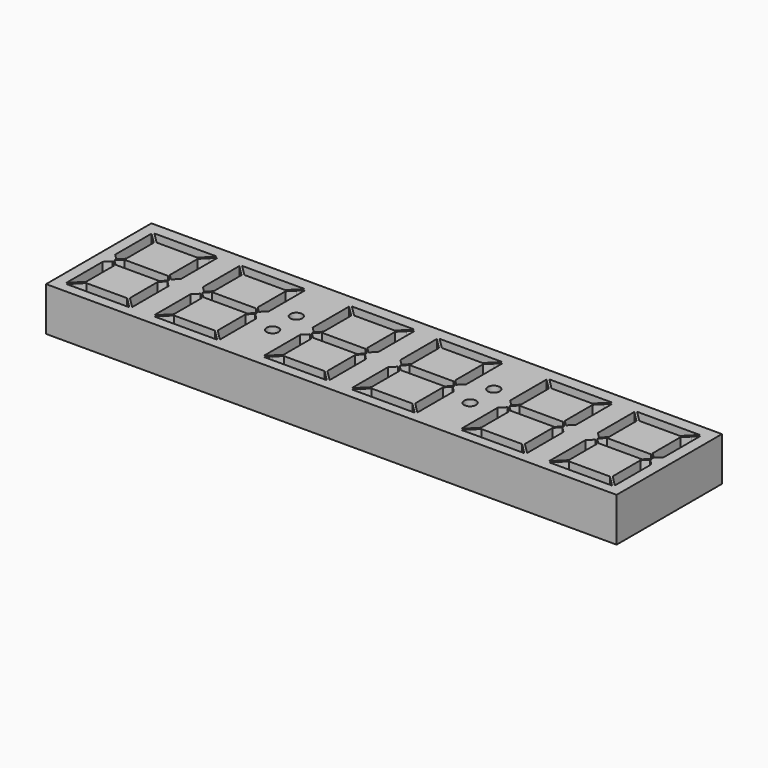
from build123d import *

# Parameters (mm, degrees)
F0_R     = 3.4648968079
F1_DEPTH = 25.4


# Not quite as in the source:
# - ends of sketch curves that miss each other by under 0.0002 mm in the source are joined


with BuildPart() as f1:
    # F0 (on Top) → F1 (new body)
    with BuildSketch(Plane.XY):
        Polygon((-45.9224169783, 52.1854245931), (-71.324658747, 52.1854245931), (-122.124658747, 52.1854245931), (-122.124658747, -24.0145754069), (-71.324658747, -24.0145754069), (-20.5201752096, -24.0145754069), (-7.824658747, -24.0145754069), (-7.8201752096, -24.0145754069), (42.975341253, -24.0145754069), (93.7798247904, -24.0145754069), (106.475341253, -24.0145754069), (106.4798247904, -24.0145754069), (157.275341253, -24.0145754069), (208.0798247904, -24.0145754069), (208.0798247904, 52.1854245931), (182.6775830217, 52.1854245931), (157.275341253, 52.1854245931), (106.4798247904, 52.1854245931), (106.475341253, 52.1854245931), (100.1298247904, 52.1854245931), (93.7798247904, 52.1854245931), (68.3775830217, 52.1854245931), (42.975341253, 52.1854245931), (-7.8201752096, 52.1854245931), (-7.824658747, 52.1854245931), (-14.1701752096, 52.1854245931), (-20.5201752096, 52.1854245931), align=None)
        Polygon((-114.8766638426, -18.2225372752), (-112.1506766486, -15.4965500813), (-108.5266638426, -11.8725372752), (-84.9227150668, -11.8725372752), (-81.2987022607, -15.4965500813), (-78.5727150668, -18.2225372752), align=None, mode=Mode.SUBTRACT)
        Polygon((-27.7726536514, -18.2225372752), (-64.0766024272, -18.2225372752), (-61.3506152332, -15.4965500813), (-57.7266024272, -11.8725372752), (-34.1226536514, -11.8725372752), (-30.4986408454, -15.4965500813), align=None, mode=Mode.SUBTRACT)
        Polygon((5.7733361574, -11.8725372752), (29.3772849332, -11.8725372752), (33.0012977393, -15.4965500813), (35.7272849332, -18.2225372752), (-0.5766638426, -18.2225372752), (2.1493233514, -15.4965500813), align=None, mode=Mode.SUBTRACT)
        Polygon((-115.7770073018, 9.0053659809), (-115.7061190955, 9.0824627244), (-112.5653735672, 12.2574627244), (-109.4246280391, 9.0824627243), (-109.4246280391, -10.9745116633), (-113.0486408451, -14.5985244694), (-115.7746284012, -17.3245116571), align=None, mode=Mode.SUBTRACT)
        Polygon((-80.8810682654, 12.2546509709), (-77.7403227372, 9.0796509709), (-77.6718137934, 9.0101770152), (-77.6718137934, -17.3273234166), (-80.3978009873, -14.6013362227), (-84.0218137919, -10.977323417), (-84.0218137936, 9.0796509708), align=None, mode=Mode.SUBTRACT)
        Polygon((-58.6275037021, -10.977323417), (-62.2515165067, -14.6013362227), (-64.9775037006, -17.3273234166), (-64.9775037006, 9.0101770152), (-64.9089947568, 9.0796509709), (-61.7682492285, 12.2546509709), (-58.6275037004, 9.0796509708), align=None, mode=Mode.SUBTRACT)
        Polygon((-112.5824693266, 13.5446828527), (-109.4275024956, 16.6996496838), (-84.0275012359, 16.699648424), (-80.866894333, 13.5446981166), (-84.0218137936, 10.349650971), (-109.4218137935, 10.349650971), (-109.4246752935, 10.3524770633), (-109.4259061434, 10.3536926829), align=None, mode=Mode.SUBTRACT)
        Polygon((-61.782423161, 13.5446981166), (-58.6218162581, 16.699648424), (-33.2218162581, 16.699648424), (-30.0668481674, 13.5446828527), (-33.2246280392, 10.3524627245), (-33.2275037004, 10.349650971), (-58.6275037003, 10.349650971), align=None, mode=Mode.SUBTRACT)
        Polygon((-26.8746890928, -17.3245116571), (-29.6006766488, -14.5985244694), (-33.2246894549, -10.9745116633), (-33.2246894549, 9.0824627243), (-30.0839439267, 12.2574627244), (-26.9431983985, 9.0824627244), (-26.8723101921, 9.0053659809), align=None, mode=Mode.SUBTRACT)
        Polygon((1.7346264327, 12.2574627244), (4.8753719609, 9.0824627243), (4.8753719609, -10.9745116633), (1.2513591549, -14.5985244694), (-1.4746284012, -17.3245116571), (-1.4770073018, 9.0053659809), (-1.4061190955, 9.0824627244), align=None, mode=Mode.SUBTRACT)
        Polygon((30.2781862081, -10.977323417), (30.2781862064, 9.0796509708), (33.4189317346, 12.2546509709), (36.5596772628, 9.0796509709), (36.6281862066, 9.0101770152), (36.6281862066, -17.3273234166), (33.9021990127, -14.6013362227), align=None, mode=Mode.SUBTRACT)
        with Locations((-14.1746894548, 4.9483692275)):
            Circle(F0_R, mode=Mode.SUBTRACT)
        Polygon((1.6986249251, 13.524648424), (1.6963722036, 13.524648424), (1.6974989639, 13.5257747847), align=None, mode=Mode.SUBTRACT)
        Polygon((4.8724987641, 16.699648424), (30.2724987641, 16.699648424), (33.4160560732, 13.5617171963), (33.433105667, 13.5446981166), (33.4503257953, 13.5621060558), (33.4503719609, 13.5274627244), (33.4160560732, 13.5274627245), (30.2781862064, 10.349650971), (4.8781862065, 10.3496509707), (4.8753105452, 10.3524627245), (1.7175306734, 13.5446828527), align=None, mode=Mode.SUBTRACT)
        Polygon((52.9493847668, -15.4965500813), (56.5733975728, -11.8725372752), (80.1773463486, -11.8725372752), (83.8013591546, -15.4965500813), (86.5273463486, -18.2225372752), (50.2233975728, -18.2225372752), align=None, mode=Mode.SUBTRACT)
        Polygon((120.0733361574, -11.8725372752), (143.6772849332, -11.8725372752), (147.3012977393, -15.4965500813), (150.0272849332, -18.2225372752), (113.7233361574, -18.2225372752), (116.4493233514, -15.4965500813), align=None, mode=Mode.SUBTRACT)
        Polygon((167.2493847668, -15.4965500813), (170.8733975728, -11.8725372752), (194.4773463486, -11.8725372752), (198.1013591546, -15.4965500813), (200.8273463486, -18.2225372752), (164.5233975728, -18.2225372752), align=None, mode=Mode.SUBTRACT)
        Polygon((52.5317507714, 12.2546509709), (55.6724962996, 9.0796509708), (55.6724962979, -10.977323417), (52.0484834933, -14.6013362227), (49.3224962994, -17.3273234166), (49.3224962994, 9.0101770152), (49.3910052432, 9.0796509709), align=None, mode=Mode.SUBTRACT)
        Polygon((81.0753105451, -10.9745116633), (81.0753105451, 9.0824627243), (84.2160560733, 12.2574627244), (87.3568016015, 9.0824627244), (87.4276898079, 9.0053659809), (87.4253109084, -17.3245116571), (84.6993233512, -14.5985244694), align=None, mode=Mode.SUBTRACT)
        Polygon((116.0346264327, 12.2574627244), (119.1753719609, 9.0824627243), (119.1753719609, -10.9745116633), (115.5513591549, -14.5985244694), (112.8253715988, -17.3245116571), (112.8229926982, 9.0053659809), (112.8938809045, 9.0824627244), align=None, mode=Mode.SUBTRACT)
        Polygon((81.0724962996, 10.3496509714), (55.6724962997, 10.3496509713), (52.5346109056, 13.5274473923), (52.5003105451, 13.5274627244), (52.5003567108, 13.5621060558), (52.517576839, 13.5446981166), (52.5346264328, 13.5617171963), (55.6781837419, 16.699648424), (81.0781837419, 16.699648424), (84.2331518326, 13.5446828527), (81.0753719608, 10.3524627245), align=None, mode=Mode.SUBTRACT)
        with Locations((100.1253105452, 4.9483692275)):
            Circle(F0_R, mode=Mode.SUBTRACT)
        Polygon((84.2531835421, 13.5257747847), (84.2543103024, 13.524648424), (84.252057581, 13.524648424), align=None, mode=Mode.SUBTRACT)
        Polygon((115.9986249251, 13.5246484235), (115.9963722036, 13.5246484235), (115.9974989639, 13.5257747847), align=None, mode=Mode.SUBTRACT)
        Polygon((144.5781862081, -10.977323417), (144.5781862064, 9.0796509708), (147.7189317346, 12.2546509709), (150.8596772628, 9.0796509709), (150.9281862066, 9.0101770152), (150.9281862066, -17.3273234166), (148.2021990127, -14.6013362227), align=None, mode=Mode.SUBTRACT)
        Polygon((166.8317507714, 12.2546509709), (169.9724962996, 9.0796509708), (169.9724962979, -10.977323417), (166.3484834933, -14.6013362227), (163.6224962994, -17.3273234166), (163.6224962994, 9.0101770152), (163.6910052432, 9.0796509709), align=None, mode=Mode.SUBTRACT)
        Polygon((195.3753105451, -10.9745116633), (195.3753105451, 9.0824627243), (198.5160560733, 12.2574627244), (201.6568016015, 9.0824627244), (201.7276898079, 9.0053659809), (201.7253109084, -17.3245116571), (198.9993233512, -14.5985244694), align=None, mode=Mode.SUBTRACT)
        Polygon((119.1724987641, 16.699648424), (144.5724987641, 16.699648424), (147.7160560732, 13.5617171963), (147.733105667, 13.5446981166), (147.7503257953, 13.5621060558), (147.7503719609, 13.5274627244), (147.7160560732, 13.5274627245), (144.5781862064, 10.349650971), (119.1781862065, 10.3496509704), (119.1753105452, 10.3524627245), (116.0175306734, 13.5446828527), align=None, mode=Mode.SUBTRACT)
        Polygon((195.3724962996, 10.3496509717), (169.9724962997, 10.3496509716), (166.8346109056, 13.5274473923), (166.8003105451, 13.5274627244), (166.8003567108, 13.5621060558), (166.817576839, 13.5446981166), (166.8346264328, 13.5617171963), (169.9781837419, 16.699648424), (195.3781837419, 16.699648424), (198.5331518326, 13.5446828527), (195.3753719608, 10.3524627245), align=None, mode=Mode.SUBTRACT)
        Polygon((198.5531835421, 13.5257747847), (198.5543103024, 13.524648424), (198.552057581, 13.5246484246), align=None, mode=Mode.SUBTRACT)
        Polygon((-112.5653735672, 14.7974627245), (-115.7061190955, 17.9724627245), (-115.7748322287, 18.0419252759), (-115.7748322287, 44.3792362755), (-113.0486408451, 41.6534499185), (-109.4246280391, 38.0294371125), (-109.4246280391, 17.9724627246), align=None, mode=Mode.SUBTRACT)
        Polygon((-77.671816009, 18.0388435052), (-77.7403866174, 17.9696484239), (-80.8839439267, 14.7974627245), (-84.0275012359, 17.969648424), (-84.0275012359, 38.0266228119), (-80.3978032029, 41.650574564), (-77.671816009, 44.376561758), align=None, mode=Mode.SUBTRACT)
        Polygon((-64.977501485, 18.0388435052), (-64.977501485, 44.376561758), (-62.251514291, 41.650574564), (-58.6218162581, 38.0266228119), (-58.6218162581, 17.969648424), (-61.7653735672, 14.7974627245), (-64.9089308765, 17.9696484239), align=None, mode=Mode.SUBTRACT)
        with Locations((-14.1746894549, 22.1065562218)):
            Circle(F0_R, mode=Mode.SUBTRACT)
        Polygon((-29.6006766488, 41.6534499185), (-26.8744852653, 44.3792362755), (-26.8744852653, 18.0419252759), (-26.9431983984, 17.9724627245), (-30.0839439267, 14.7974627245), (-33.2246894549, 17.9724627246), (-33.2246894549, 38.0294371125), align=None, mode=Mode.SUBTRACT)
        Polygon((-1.4748322287, 18.0419252759), (-1.4748322287, 44.3792359067), (1.2513591549, 41.6534499185), (4.8753719609, 38.0294371125), (4.8753719609, 17.9724627246), (1.7346264328, 14.7974627245), (-1.4061190955, 17.9724627245), align=None, mode=Mode.SUBTRACT)
        Polygon((30.2724987641, 17.969648424), (30.2724987641, 38.0266228119), (33.9021967971, 41.650574564), (36.628183991, 44.376561758), (36.628183991, 18.0388435052), (36.5596133826, 17.9696484239), (33.4160560733, 14.7974627245), align=None, mode=Mode.SUBTRACT)
        Polygon((-78.572653651, 45.2774627244), (-81.298640845, 42.5514755305), (-84.9226536512, 38.9274627246), (-108.526602427, 38.9274627246), (-112.150615233, 42.5514755306), (-114.8766024268, 45.2774627244), align=None, mode=Mode.SUBTRACT)
        Polygon((-61.350676649, 42.5514755305), (-64.0766638429, 45.2774627244), (-27.7727150671, 45.2774627244), (-30.4987022609, 42.5514755306), (-34.122715067, 38.9274627246), (-57.7266638428, 38.9274627246), align=None, mode=Mode.SUBTRACT)
        Polygon((-0.5766024268, 45.2774627244), (35.727346349, 45.2774627244), (33.001359155, 42.5514755305), (29.3773463488, 38.9274627246), (5.773397573, 38.9274627246), (2.149384767, 42.5514755306), align=None, mode=Mode.SUBTRACT)
        with Locations((100.1253105451, 22.1065562218)):
            Circle(F0_R, mode=Mode.SUBTRACT)
        Polygon((49.322498515, 18.0388435052), (49.322498515, 44.376561758), (52.048485709, 41.650574564), (55.6781837419, 38.0266228119), (55.6781837419, 17.969648424), (52.5346264328, 14.7974627245), (49.3910691235, 17.9696484239), align=None, mode=Mode.SUBTRACT)
        Polygon((84.6993233512, 41.6534499185), (87.4255147347, 44.3792362755), (87.4255147347, 18.0419252759), (87.3568016016, 17.9724627245), (84.2160560733, 14.7974627245), (81.0753105451, 17.9724627246), (81.0753105451, 38.0294371125), align=None, mode=Mode.SUBTRACT)
        Polygon((112.8251677713, 18.0419252759), (112.8251677713, 44.3792359067), (115.5513591549, 41.6534499185), (119.1753719609, 38.0294371125), (119.1753719609, 17.9724627246), (116.0346264328, 14.7974627245), (112.8938809045, 17.9724627245), align=None, mode=Mode.SUBTRACT)
        Polygon((144.5724987641, 17.969648424), (144.5724987641, 38.0266228119), (148.2021967971, 41.650574564), (150.928183991, 44.376561758), (150.928183991, 18.0388435052), (150.8596133826, 17.9696484239), (147.7160560733, 14.7974627245), align=None, mode=Mode.SUBTRACT)
        Polygon((163.622498515, 18.0388435052), (163.622498515, 44.376561758), (166.348485709, 41.650574564), (169.9781837419, 38.0266228119), (169.9781837419, 17.969648424), (166.8346264328, 14.7974627245), (163.6910691235, 17.9696484239), align=None, mode=Mode.SUBTRACT)
        Polygon((198.9993233512, 41.6534499185), (201.7255147347, 44.3792362755), (201.7255147347, 18.0419252759), (201.6568016016, 17.9724627245), (198.5160560733, 14.7974627245), (195.3753105451, 17.9724627246), (195.3753105451, 38.0294371125), align=None, mode=Mode.SUBTRACT)
        Polygon((80.177284933, 38.9274627246), (56.5733361572, 38.9274627246), (52.949323351, 42.5514755305), (50.2233361571, 45.2774627244), (86.5272849329, 45.2774627244), (83.8012977391, 42.5514755306), align=None, mode=Mode.SUBTRACT)
        Polygon((113.7233975732, 45.2774627244), (150.027346349, 45.2774627244), (147.301359155, 42.5514755305), (143.6773463488, 38.9274627246), (120.073397573, 38.9274627246), (116.449384767, 42.5514755306), align=None, mode=Mode.SUBTRACT)
        Polygon((194.477284933, 38.9274627246), (170.8733361572, 38.9274627246), (167.249323351, 42.5514755305), (164.5233361571, 45.2774627244), (200.8272849329, 45.2774627244), (198.1012977391, 42.5514755306), align=None, mode=Mode.SUBTRACT)
    extrude(amount=F1_DEPTH)


solid = f1.part
